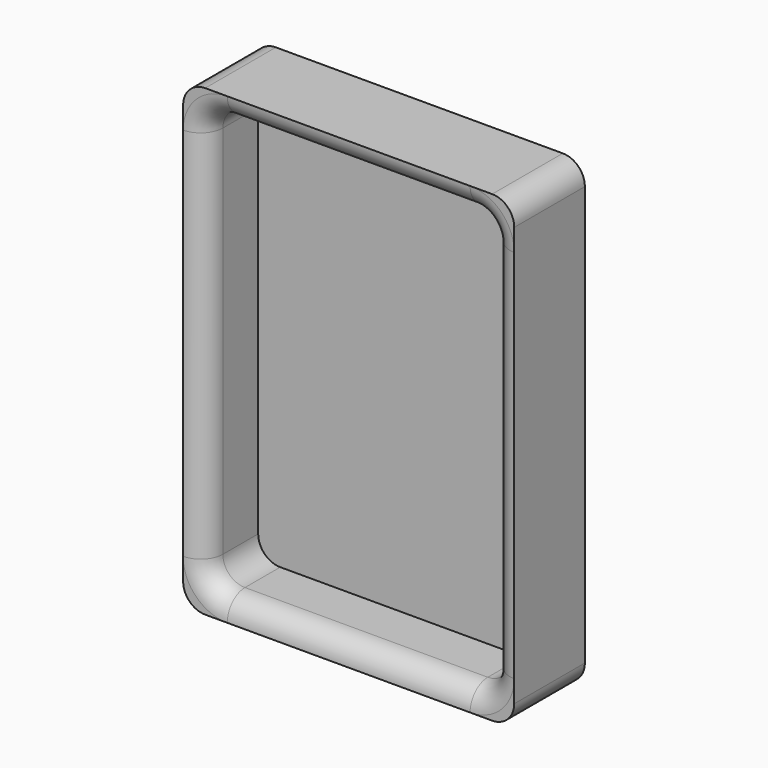
from build123d import *

# Parameters (mm, degrees)
F0_W     = 75
F0_H     = 105
F1_DEPTH = 20
F2_T     = -5
F3_R     = 5
F3_R_2   = 4.99999


# Not quite as in the source:
# - a fillet or chamfer is up to 0.001 mm smaller than in the source, because OpenCascade refuses the exact size


with BuildPart() as f1:
    # F0 (on Front) → F1 (new body)
    with BuildSketch(Plane.XZ):
        with Locations((0.4762494937, 1.3404280991)):
            Rectangle(F0_W, F0_H)
    extrude(amount=F1_DEPTH)

    # F2
    f2_openings = [f1.faces().sort_by_distance(p)[0] for p in [
        (0.476249, -20, 1.340428),
    ]]
    offset(amount=F2_T, openings=f2_openings)

    # F3 (call 1 of 5: OpenCascade refuses the feature's edges together)
    f3_edges = [f1.edges().sort_by_distance(p)[0] for p in [
        (-37.023751, -10, 53.840428),
    ]]
    fillet(f3_edges, radius=F3_R)

    # F3#2 (call 2 of 5)
    f3_2_edges = [f1.edges().sort_by_distance(p)[0] for p in [
        (-37.023751, -10, -51.159572),
    ]]
    fillet(f3_2_edges, radius=F3_R)

    # F3#3 (call 3 of 5)
    f3_3_edges = [f1.edges().sort_by_distance(p)[0] for p in [
        (37.976249, -10, 53.840428),
    ]]
    fillet(f3_3_edges, radius=F3_R)

    # F3#4 (call 4 of 5)
    f3_4_edges = [f1.edges().sort_by_distance(p)[0] for p in [
        (37.976249, -10, -51.159572),
    ]]
    fillet(f3_4_edges, radius=F3_R)

    # F3#5 (call 5 of 5) (radius 5 in the source; OpenCascade refuses exactly that, so slightly less here)
    f3_5_edges = [f1.edges().sort_by_distance(p)[0] for p in [
        (-32.023751, -12.5, 48.840428),
        (32.976249, -12.5, 48.840428),
        (-32.023751, -12.5, -46.159572),
        (32.976249, -12.5, -46.159572),
        (32.976249, -20, 1.340428),
        (-32.023751, -20, 1.340428),
        (0.476249, -20, 48.840428),
        (0.476249, -20, -46.159572),
    ]]
    fillet(f3_5_edges, radius=F3_R_2)


solid = f1.part
